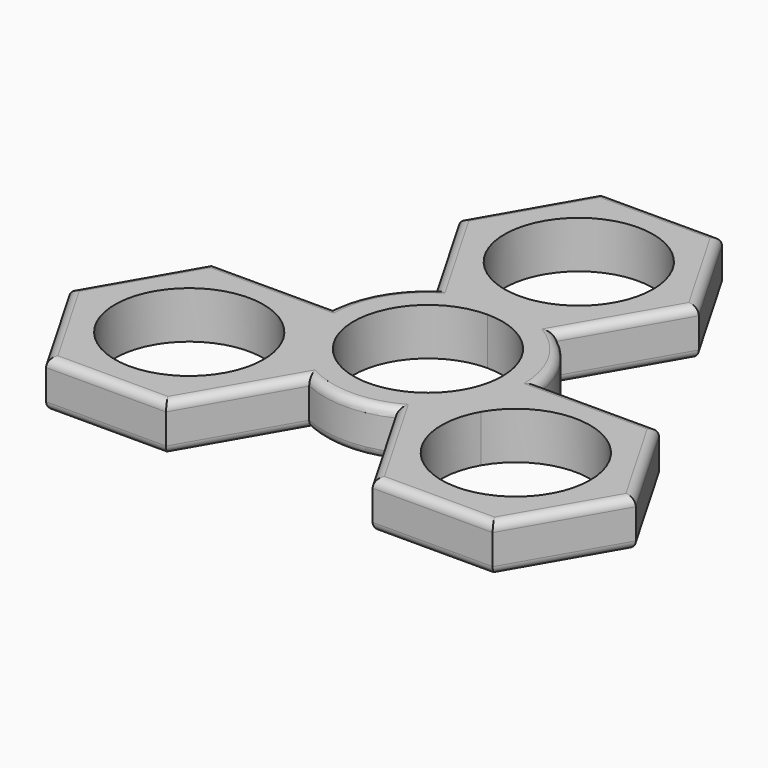
from build123d import *

# Parameters (mm, degrees)
F1_DEPTH      = 6.985
F2_T3_DEPTH   = 24.13
F2_S4_R       = 15.3732097417
F2_T5_DEPTH   = 14
F2_T8_DEPTH   = 24.13
F2_T11_DEPTH  = 24.13
F2_T14_DEPTH  = 24.13
F2_T17_DEPTH  = 24.13
F2_S18_R      = 15.3732097417
F2_T19_DEPTH  = 14
F2_T22_ANGLE  = 73.0101001262
F2_T27_ANGLE  = 73.0101001262
F2_T32_DEPTH  = 24.13
F2_S33_R      = 15.3732097417
F2_T34_DEPTH  = 14
F2_T37_DEPTH  = 24.13
F2_T40_DEPTH  = 24.13
F2_T43_DEPTH  = 24.13
F2_T46_ANGLE  = 73.0101001262
F2_T51_DEPTH  = 24.13
F2_S52_R      = 15.3732097417
F2_T53_DEPTH  = 14
F2_T56_DEPTH  = 24.13
F2_T59_DEPTH  = 24.13
F2_T62_DEPTH  = 24.13
F2_T65_DEPTH  = 24.13
F2_S66_R      = 15.3732097417
F2_T67_DEPTH  = 14
F2_T70_DEPTH  = 24.13
F2_S71_R      = 15.3732097417
F2_T72_DEPTH  = 14
F2_T76_DEPTH  = 24.13
F2_S77_R      = 15.3732097417
F2_T78_DEPTH  = 14
F2_T81_ANGLE  = 73.0101001262
F2_T87_DEPTH  = 24.13
F2_S88_R      = 15.3732097417
F2_T89_DEPTH  = 14
F2_T92_ANGLE  = 73.0101001262
F2_T98_DEPTH  = 24.13
F2_S99_R      = 15.3732097417
F2_T100_DEPTH = 14
F2_T103_ANGLE = 73.0101001262
F2_T109_ANGLE = 73.0101001262
F2_T113_DEPTH = 24.13
F2_S114_R     = 15.3732097417
F2_T115_DEPTH = 14
F2_T120_DEPTH = 24.13
F2_S121_R     = 15.3732097417
F2_T122_DEPTH = 14
F2_T125_ANGLE = 73.0101001262
F2_T131_ANGLE = 73.0101001262
F2_T135_DEPTH = 24.13
F2_S136_R     = 15.3732097417
F2_T137_DEPTH = 14
F3_R          = 1.27


# Not quite as in the source:
# - a fillet or chamfer that OpenCascade refuses, or shapes differently, is made with other operations: its cross-section is extruded or revolved along the edge and cut away or added


with BuildPart() as f1:
    # F0 (on Top) → F1 (new body)
    with BuildSketch(Plane.XY):
        with BuildLine():
            ThreePointArc((0, 11.0109), (7.785882057, 7.785882057), (11.0109, 0))
            ThreePointArc((11.0109, 0), (10.6357126807, -2.8498306237), (9.5357191185, -5.50545))
            Line((9.5357191185, -5.50545), (10.8617497817, -6.2710341604))
            Line((10.8617497817, -6.2710341604), (15.3067497817, 1.4279316793))
            ThreePointArc((15.3067497817, 1.4279316793), (13.313590174, 7.6866048708), (8.89, 12.5420683207))
            Line((8.89, 12.5420683207), (0, 12.5420683207))
            Line((0, 12.5420683207), (0, 11.0109))
        make_face()
        with BuildLine():
            ThreePointArc((-9.5357191185, -5.50545), (-9.5357191185, 5.50545), (0, 11.0109))
            Line((0, 11.0109), (0, 12.5420683207))
            Line((0, 12.5420683207), (-8.89, 12.5420683207))
            ThreePointArc((-8.89, 12.5420683207), (-13.313590174, 7.6866048708), (-15.3067497817, 1.4279316793))
            Line((-15.3067497817, 1.4279316793), (-10.8617497817, -6.2710341604))
            Line((-10.8617497817, -6.2710341604), (-9.5357191185, -5.50545))
        make_face()
        with BuildLine():
            Line((10.8617497817, -6.2710341604), (9.5357191185, -5.50545))
            ThreePointArc((9.5357191185, -5.50545), (0, -11.0109), (-9.5357191185, -5.50545))
            Line((-9.5357191185, -5.50545), (-10.8617497817, -6.2710341604))
            Line((-10.8617497817, -6.2710341604), (-6.4167497817, -13.97))
            ThreePointArc((-6.4167497817, -13.97), (0, -15.3732097417), (6.4167497817, -13.97))
            Line((6.4167497817, -13.97), (10.8617497817, -6.2710341604))
        make_face()
        with BuildLine():
            Line((-8.89, 12.5420683207), (0, 12.5420683207))
            Line((0, 12.5420683207), (0, 15.3732097417))
            ThreePointArc((0, 15.3732097417), (-4.6649614614, 14.648334797), (-8.89, 12.5420683207))
        make_face()
        with BuildLine():
            Line((0, 15.3732097417), (0, 12.5420683207))
            Line((0, 12.5420683207), (8.89, 12.5420683207))
            ThreePointArc((8.89, 12.5420683207), (4.6649614614, 14.648334797), (0, 15.3732097417))
        make_face()
        with BuildLine():
            Line((15.3067497817, 1.4279316793), (10.8617497817, -6.2710341604))
            Line((10.8617497817, -6.2710341604), (13.313590174, -7.6866048708))
            ThreePointArc((13.313590174, -7.6866048708), (14.8493803224, -3.9788794655), (15.3732097417, 0))
            ThreePointArc((15.3732097417, 0), (15.3565857634, 0.7147387297), (15.3067497817, 1.4279316793))
        make_face()
        with BuildLine():
            Line((13.313590174, -7.6866048708), (10.8617497817, -6.2710341604))
            Line((10.8617497817, -6.2710341604), (6.4167497817, -13.97))
            ThreePointArc((6.4167497817, -13.97), (10.3533493266, -11.3641425318), (13.313590174, -7.6866048708))
        make_face()
        with BuildLine():
            Line((-6.4167497817, -13.97), (-10.8617497817, -6.2710341604))
            Line((-10.8617497817, -6.2710341604), (-13.313590174, -7.6866048708))
            ThreePointArc((-13.313590174, -7.6866048708), (-10.3533493266, -11.3641425318), (-6.4167497817, -13.97))
        make_face()
        with BuildLine():
            Line((-13.313590174, -7.6866048708), (-10.8617497817, -6.2710341604))
            Line((-10.8617497817, -6.2710341604), (-15.3067497817, 1.4279316793))
            ThreePointArc((-15.3067497817, 1.4279316793), (-15.018310788, -3.2841922653), (-13.313590174, -7.6866048708))
        make_face()
        with BuildLine():
            ThreePointArc((-8.89, 12.5420683207), (-4.6649614614, 14.648334797), (0, 15.3732097417))
            ThreePointArc((0, 15.3732097417), (4.6649614614, 14.648334797), (8.89, 12.5420683207))
            Line((8.89, 12.5420683207), (17.78, 27.94))
            Line((17.78, 27.94), (8.89, 43.3379316793))
            Line((8.89, 43.3379316793), (-8.89, 43.3379316793))
            Line((-8.89, 43.3379316793), (-17.78, 27.94))
            Line((-17.78, 27.94), (-8.89, 12.5420683207))
        make_face()
        with BuildLine():
            ThreePointArc((11.0109, 27.94), (7.785882057, 20.154117943), (0, 16.9291))
            ThreePointArc((0, 16.9291), (-7.785882057, 35.725882057), (11.0109, 27.94))
        make_face(mode=Mode.SUBTRACT)
        with BuildLine():
            ThreePointArc((15.3732097417, 0), (14.8493803224, -3.9788794655), (13.313590174, -7.6866048708))
            ThreePointArc((13.313590174, -7.6866048708), (10.3533493266, -11.3641425318), (6.4167497817, -13.97))
            Line((6.4167497817, -13.97), (15.3067497817, -29.3679316793))
            Line((15.3067497817, -29.3679316793), (33.0867497817, -29.3679316793))
            Line((33.0867497817, -29.3679316793), (41.9767497817, -13.97))
            Line((41.9767497817, -13.97), (33.0867497817, 1.4279316793))
            Line((33.0867497817, 1.4279316793), (15.3067497817, 1.4279316793))
            ThreePointArc((15.3067497817, 1.4279316793), (15.3565857634, 0.7147387297), (15.3732097417, 0))
        make_face()
        with BuildLine():
            ThreePointArc((35.2076497817, -13.97), (21.346919158, -24.6057126807), (14.6610306632, -8.46455))
            ThreePointArc((14.6610306632, -8.46455), (27.0465804055, -3.3342873193), (35.2076497817, -13.97))
        make_face(mode=Mode.SUBTRACT)
        with BuildLine():
            ThreePointArc((-6.4167497817, -13.97), (-10.3533493266, -11.3641425318), (-13.313590174, -7.6866048708))
            ThreePointArc((-13.313590174, -7.6866048708), (-15.018310788, -3.2841922653), (-15.3067497817, 1.4279316793))
            Line((-15.3067497817, 1.4279316793), (-33.0867497817, 1.4279316793))
            Line((-33.0867497817, 1.4279316793), (-41.9767497817, -13.97))
            Line((-41.9767497817, -13.97), (-33.0867497817, -29.3679316793))
            Line((-33.0867497817, -29.3679316793), (-15.3067497817, -29.3679316793))
            Line((-15.3067497817, -29.3679316793), (-6.4167497817, -13.97))
        make_face()
        with BuildLine():
            ThreePointArc((-13.1858497817, -13.97), (-34.8324624624, -16.8198306237), (-14.6610306632, -8.46455))
            ThreePointArc((-14.6610306632, -8.46455), (-13.5610371011, -11.1201693763), (-13.1858497817, -13.97))
        make_face(mode=Mode.SUBTRACT)
    extrude(amount=F1_DEPTH)

    # F2: fillet of radius 1.27 on 18 edges, made by hand


with BuildPart() as f2_tool1:
    # F2_s2 → F2_t3 (new body)
    with BuildSketch(Plane(origin=(-18.1308748909, 31.4035964967, 0), x_dir=(0, 0, 1), z_dir=(0.5, -0.8660254038, 0))):
        with BuildLine():
            ThreePointArc((5.715, 1.4279316793), (6.6130256121, 1.0559572914), (6.985, 0.1579316793))
            Line((6.985, 0.1579316793), (6.985, 1.4279316793))
            Line((6.985, 1.4279316793), (5.715, 1.4279316793))
        make_face()
    extrude(amount=F2_T3_DEPTH)

    # F2_s4 → F2_t5 (cut, symmetric)
    with BuildSketch(Plane.XY.offset(6.4)):
        Circle(F2_S4_R)
    extrude(amount=F2_T5_DEPTH, both=True, mode=Mode.SUBTRACT)


with BuildPart() as f2_tool6:
    # F2_s7 → F2_t8 (new body)
    with BuildSketch(Plane(origin=(18.1308748909, 31.4035964967, 0), x_dir=(0, 0, 1), z_dir=(-0.5, -0.8660254038, 0))):
        with BuildLine():
            ThreePointArc((5.715, 29.3679316793), (6.6130256121, 28.9959572914), (6.985, 28.0979316793))
            Line((6.985, 28.0979316793), (6.985, 29.3679316793))
            Line((6.985, 29.3679316793), (5.715, 29.3679316793))
        make_face()
    extrude(amount=F2_T8_DEPTH)


with BuildPart() as f2_tool9:
    # F2_s10 → F2_t11 (new body)
    with BuildSketch(Plane.YZ.offset(12.065)):
        with BuildLine():
            ThreePointArc((43.3379316793, 5.715), (42.9659572914, 6.6130256121), (42.0679316793, 6.985))
            Line((42.0679316793, 6.985), (43.3379316793, 6.985))
            Line((43.3379316793, 6.985), (43.3379316793, 5.715))
        make_face()
    extrude(amount=-F2_T11_DEPTH)


with BuildPart() as f2_tool12:
    # F2_s13 → F2_t14 (new body)
    with BuildSketch(Plane(origin=(-6.0658748909, 10.5064035033, 0), x_dir=(0, 0, 1), z_dir=(-0.5, 0.8660254038, 0))):
        with BuildLine():
            ThreePointArc((5.715, 29.3679316793), (6.6130256121, 28.9959572914), (6.985, 28.0979316793))
            Line((6.985, 28.0979316793), (6.985, 29.3679316793))
            Line((6.985, 29.3679316793), (5.715, 29.3679316793))
        make_face()
    extrude(amount=F2_T14_DEPTH)


with BuildPart() as f2_tool15:
    # F2_s16 → F2_t17 (new body)
    with BuildSketch(Plane(origin=(6.0658748909, 10.5064035033, 0), x_dir=(0, 0, 1), z_dir=(0.5, 0.8660254038, 0))):
        with BuildLine():
            ThreePointArc((5.715, 1.4279316793), (6.6130256121, 1.0559572914), (6.985, 0.1579316793))
            Line((6.985, 0.1579316793), (6.985, 1.4279316793))
            Line((6.985, 1.4279316793), (5.715, 1.4279316793))
        make_face()
    extrude(amount=F2_T17_DEPTH)

    # F2_s18 → F2_t19 (cut, symmetric)
    with BuildSketch(Plane.XY.offset(6.4)):
        Circle(F2_S18_R)
    extrude(amount=F2_T19_DEPTH, both=True, mode=Mode.SUBTRACT)


with BuildPart() as f2_tool20:
    # F2_s21 → F2_t22 (revolve)
    with BuildSketch(Plane(origin=(0, 0, 0), x_dir=(0, 0, 1), z_dir=(-0.113290787, -0.9935618741, 0))):
        with BuildLine():
            ThreePointArc((5.715, -15.3732097417), (6.6130256121, -15.0012353538), (6.985, -14.1032097417))
            Line((6.985, -14.1032097417), (6.985, -15.3732097417))
            Line((6.985, -15.3732097417), (5.715, -15.3732097417))
        make_face()
    revolve(axis=Axis((0, 0, 6.985), (0, 0, 1)), revolution_arc=F2_T22_ANGLE)

    split(bisect_by=Plane(origin=(1.2366251091, -0.7139658396, 0), x_dir=(0, 0, 1), z_dir=(0.8660254038, -0.5, 0)), keep=Keep.TOP)

    split(bisect_by=Plane.XZ.offset(-1.4279316793), keep=Keep.BOTTOM)


with BuildPart() as f2_tool25:
    # F2_s26 → F2_t27 (revolve)
    with BuildSketch(Plane(origin=(0, 0, 0), x_dir=(0, 0, 1), z_dir=(0.9170952167, 0.3986682375, 0))):
        with BuildLine():
            ThreePointArc((5.715, -15.3732097417), (6.6130256121, -15.0012353538), (6.985, -14.1032097417))
            Line((6.985, -14.1032097417), (6.985, -15.3732097417))
            Line((6.985, -15.3732097417), (5.715, -15.3732097417))
        make_face()
    revolve(axis=Axis((0, 0, 6.985), (0, 0, 1)), revolution_arc=F2_T27_ANGLE)

    split(bisect_by=Plane(origin=(-1.2366251091, -0.7139658396, 0), x_dir=(0, 0, 1), z_dir=(-0.8660254038, -0.5, 0)), keep=Keep.TOP)

    split(bisect_by=Plane.XZ.offset(-1.4279316793), keep=Keep.BOTTOM)


with BuildPart() as f2_tool30:
    # F2_s31 → F2_t32 (new body)
    with BuildSketch(Plane.YZ.offset(-12.1317497817)):
        with BuildLine():
            ThreePointArc((1.4279316793, 5.715), (1.0559572914, 6.6130256121), (0.1579316793, 6.985))
            Line((0.1579316793, 6.985), (1.4279316793, 6.985))
            Line((1.4279316793, 6.985), (1.4279316793, 5.715))
        make_face()
    extrude(amount=-F2_T32_DEPTH)

    # F2_s33 → F2_t34 (cut, symmetric)
    with BuildSketch(Plane.XY.offset(6.4)):
        Circle(F2_S33_R)
    extrude(amount=F2_T34_DEPTH, both=True, mode=Mode.SUBTRACT)


with BuildPart() as f2_tool35:
    # F2_s36 → F2_t37 (new body)
    with BuildSketch(Plane(origin=(-6.0658748909, -10.5064035033, 0), x_dir=(0, 0, 1), z_dir=(-0.5, -0.8660254038, 0))):
        with BuildLine():
            ThreePointArc((5.715, 29.3679316793), (6.6130256121, 28.9959572914), (6.985, 28.0979316793))
            Line((6.985, 28.0979316793), (6.985, 29.3679316793))
            Line((6.985, 29.3679316793), (5.715, 29.3679316793))
        make_face()
    extrude(amount=F2_T37_DEPTH)


with BuildPart() as f2_tool38:
    # F2_s39 → F2_t40 (new body)
    with BuildSketch(Plane(origin=(-6.0325, 10.4485964967, 0), x_dir=(0, 0, 1), z_dir=(0.5, -0.8660254038, 0))):
        with BuildLine():
            ThreePointArc((5.715, 43.3379316793), (6.6130256121, 42.9659572914), (6.985, 42.0679316793))
            Line((6.985, 42.0679316793), (6.985, 43.3379316793))
            Line((6.985, 43.3379316793), (5.715, 43.3379316793))
        make_face()
    extrude(amount=F2_T40_DEPTH)


with BuildPart() as f2_tool41:
    # F2_s42 → F2_t43 (new body)
    with BuildSketch(Plane.YZ.offset(-36.2617497817)):
        with BuildLine():
            ThreePointArc((-29.3679316793, 5.715), (-28.9959572914, 6.6130256121), (-28.0979316793, 6.985))
            Line((-28.0979316793, 6.985), (-29.3679316793, 6.985))
            Line((-29.3679316793, 6.985), (-29.3679316793, 5.715))
        make_face()
    extrude(amount=F2_T43_DEPTH)


with BuildPart() as f2_tool44:
    # F2_s45 → F2_t46 (revolve)
    with BuildSketch(Plane(origin=(0, 0, 0), x_dir=(0, 0, 1), z_dir=(-0.8038044297, 0.5948936366, 0))):
        with BuildLine():
            ThreePointArc((5.715, -15.3732097417), (6.6130256121, -15.0012353538), (6.985, -14.1032097417))
            Line((6.985, -14.1032097417), (6.985, -15.3732097417))
            Line((6.985, -15.3732097417), (5.715, -15.3732097417))
        make_face()
    revolve(axis=Axis((0, 0, 6.985), (0, 0, 1)), revolution_arc=F2_T46_ANGLE)

    split(bisect_by=Plane(origin=(1.2366251091, -0.7139658396, 0), x_dir=(0, 0, 1), z_dir=(0.8660254038, -0.5, 0)), keep=Keep.TOP)

    split(bisect_by=Plane(origin=(-1.2366251091, -0.7139658396, 0), x_dir=(0, 0, 1), z_dir=(-0.8660254038, -0.5, 0)), keep=Keep.TOP)


with BuildPart() as f2_tool49:
    # F2_s50 → F2_t51 (new body)
    with BuildSketch(Plane(origin=(6.0658748909, -10.5064035033, 0), x_dir=(0, 0, 1), z_dir=(0.5, -0.8660254038, 0))):
        with BuildLine():
            ThreePointArc((5.715, 1.4279316793), (6.6130256121, 1.0559572914), (6.985, 0.1579316793))
            Line((6.985, 0.1579316793), (6.985, 1.4279316793))
            Line((6.985, 1.4279316793), (5.715, 1.4279316793))
        make_face()
    extrude(amount=F2_T51_DEPTH)

    # F2_s52 → F2_t53 (cut, symmetric)
    with BuildSketch(Plane.XY.offset(6.4)):
        Circle(F2_S52_R)
    extrude(amount=F2_T53_DEPTH, both=True, mode=Mode.SUBTRACT)


with BuildPart() as f2_tool54:
    # F2_s55 → F2_t56 (new body)
    with BuildSketch(Plane.YZ.offset(12.1317497817)):
        with BuildLine():
            ThreePointArc((-29.3679316793, 5.715), (-28.9959572914, 6.6130256121), (-28.0979316793, 6.985))
            Line((-28.0979316793, 6.985), (-29.3679316793, 6.985))
            Line((-29.3679316793, 6.985), (-29.3679316793, 5.715))
        make_face()
    extrude(amount=F2_T56_DEPTH)


with BuildPart() as f2_tool57:
    # F2_s58 → F2_t59 (new body)
    with BuildSketch(Plane(origin=(-6.0325, -10.4485964967, 0), x_dir=(0, 0, 1), z_dir=(0.5, 0.8660254038, 0))):
        with BuildLine():
            ThreePointArc((5.715, 43.3379316793), (6.6130256121, 42.9659572914), (6.985, 42.0679316793))
            Line((6.985, 42.0679316793), (6.985, 43.3379316793))
            Line((6.985, 43.3379316793), (5.715, 43.3379316793))
        make_face()
    extrude(amount=F2_T59_DEPTH)


with BuildPart() as f2_tool60:
    # F2_s61 → F2_t62 (new body)
    with BuildSketch(Plane(origin=(18.1308748909, -31.4035964967, 0), x_dir=(0, 0, 1), z_dir=(-0.5, 0.8660254038, 0))):
        with BuildLine():
            ThreePointArc((5.715, 29.3679316793), (6.6130256121, 28.9959572914), (6.985, 28.0979316793))
            Line((6.985, 28.0979316793), (6.985, 29.3679316793))
            Line((6.985, 29.3679316793), (5.715, 29.3679316793))
        make_face()
    extrude(amount=F2_T62_DEPTH)


with BuildPart() as f2_tool63:
    # F2_s64 → F2_t65 (new body)
    with BuildSketch(Plane.YZ.offset(36.2617497817)):
        with BuildLine():
            ThreePointArc((1.4279316793, 5.715), (1.0559572914, 6.6130256121), (0.1579316793, 6.985))
            Line((0.1579316793, 6.985), (1.4279316793, 6.985))
            Line((1.4279316793, 6.985), (1.4279316793, 5.715))
        make_face()
    extrude(amount=-F2_T65_DEPTH)

    # F2_s66 → F2_t67 (cut, symmetric)
    with BuildSketch(Plane.XY.offset(6.4)):
        Circle(F2_S66_R)
    extrude(amount=F2_T67_DEPTH, both=True, mode=Mode.SUBTRACT)


with BuildPart() as f2_tool68:
    # F2_s69 → F2_t70 (new body)
    with BuildSketch(Plane(origin=(-18.1308748909, -31.4035964967, 0), x_dir=(0, 0, 1), z_dir=(0.5, 0.8660254038, 0))):
        with BuildLine():
            ThreePointArc((5.715, 1.4279316793), (6.6130256121, 1.0559572914), (6.985, 0.1579316793))
            Line((6.985, 0.1579316793), (6.985, 1.4279316793))
            Line((6.985, 1.4279316793), (5.715, 1.4279316793))
        make_face()
    extrude(amount=F2_T70_DEPTH)

    # F2_s71 → F2_t72 (cut, symmetric)
    with BuildSketch(Plane.XY.offset(6.4)):
        Circle(F2_S71_R)
    extrude(amount=F2_T72_DEPTH, both=True, mode=Mode.SUBTRACT)


with BuildPart() as f2_tool74:
    # F2_s75 → F2_t76 (new body)
    with BuildSketch(Plane(origin=(-18.1308748909, 31.4035964967, 0), x_dir=(0, 0, 1), z_dir=(0.5, -0.8660254038, 0))):
        with BuildLine():
            ThreePointArc((5.715, 1.4279316793), (6.6130256121, 1.0559572914), (6.985, 0.1579316793))
            Line((6.985, 0.1579316793), (6.985, 1.4279316793))
            Line((6.985, 1.4279316793), (5.715, 1.4279316793))
        make_face()
    extrude(amount=F2_T76_DEPTH)

    # F2_s77 → F2_t78 (intersect, symmetric)
    with BuildSketch(Plane.XY.offset(6.4)):
        Circle(F2_S77_R)
    extrude(amount=F2_T78_DEPTH, both=True, mode=Mode.INTERSECT)


with BuildPart() as f2_tool79:
    # F2_s80 → F2_t81 (revolve)
    with BuildSketch(Plane(origin=(0, 0, 0), x_dir=(0, 0, 1), z_dir=(0.9170952167, 0.3986682375, 0))):
        with BuildLine():
            ThreePointArc((5.715, -15.3732097417), (6.6130256121, -15.0012353538), (6.985, -14.1032097417))
            Line((6.985, -14.1032097417), (6.985, -15.3732097417))
            Line((6.985, -15.3732097417), (5.715, -15.3732097417))
        make_face()
    revolve(axis=Axis((0, 0, 6.985), (0, 0, 1)), revolution_arc=F2_T81_ANGLE)

    split(bisect_by=Plane(origin=(-1.2366251091, -0.7139658396, 0), x_dir=(0, 0, 1), z_dir=(0.8660254038, 0.5, 0)), keep=Keep.TOP)


with BuildPart() as f2_tool74_1:
    add(f2_tool74.part)

    # F2_t83: intersect F2_tool79
    add(f2_tool79.part, mode=Mode.INTERSECT)


with BuildPart() as f2_tool85:
    # F2_s86 → F2_t87 (new body)
    with BuildSketch(Plane(origin=(6.0658748909, 10.5064035033, 0), x_dir=(0, 0, 1), z_dir=(0.5, 0.8660254038, 0))):
        with BuildLine():
            ThreePointArc((5.715, 1.4279316793), (6.6130256121, 1.0559572914), (6.985, 0.1579316793))
            Line((6.985, 0.1579316793), (6.985, 1.4279316793))
            Line((6.985, 1.4279316793), (5.715, 1.4279316793))
        make_face()
    extrude(amount=F2_T87_DEPTH)

    # F2_s88 → F2_t89 (intersect, symmetric)
    with BuildSketch(Plane.XY.offset(6.4)):
        Circle(F2_S88_R)
    extrude(amount=F2_T89_DEPTH, both=True, mode=Mode.INTERSECT)


with BuildPart() as f2_tool90:
    # F2_s91 → F2_t92 (revolve)
    with BuildSketch(Plane(origin=(0, 0, 0), x_dir=(0, 0, 1), z_dir=(-0.113290787, -0.9935618741, 0))):
        with BuildLine():
            ThreePointArc((5.715, -15.3732097417), (6.6130256121, -15.0012353538), (6.985, -14.1032097417))
            Line((6.985, -14.1032097417), (6.985, -15.3732097417))
            Line((6.985, -15.3732097417), (5.715, -15.3732097417))
        make_face()
    revolve(axis=Axis((0, 0, 6.985), (0, 0, 1)), revolution_arc=F2_T92_ANGLE)

    split(bisect_by=Plane(origin=(1.2366251091, -0.7139658396, 0), x_dir=(0, 0, 1), z_dir=(-0.8660254038, 0.5, 0)), keep=Keep.TOP)


with BuildPart() as f2_tool85_1:
    add(f2_tool85.part)

    # F2_t94: intersect F2_tool90
    add(f2_tool90.part, mode=Mode.INTERSECT)


with BuildPart() as f2_tool96:
    # F2_s97 → F2_t98 (new body)
    with BuildSketch(Plane.YZ.offset(36.2617497817)):
        with BuildLine():
            ThreePointArc((1.4279316793, 5.715), (1.0559572914, 6.6130256121), (0.1579316793, 6.985))
            Line((0.1579316793, 6.985), (1.4279316793, 6.985))
            Line((1.4279316793, 6.985), (1.4279316793, 5.715))
        make_face()
    extrude(amount=-F2_T98_DEPTH)

    # F2_s99 → F2_t100 (intersect, symmetric)
    with BuildSketch(Plane.XY.offset(6.4)):
        Circle(F2_S99_R)
    extrude(amount=F2_T100_DEPTH, both=True, mode=Mode.INTERSECT)


with BuildPart() as f2_tool101:
    # F2_s102 → F2_t103 (revolve)
    with BuildSketch(Plane(origin=(0, 0, 0), x_dir=(0, 0, 1), z_dir=(-0.113290787, -0.9935618741, 0))):
        with BuildLine():
            ThreePointArc((5.715, -15.3732097417), (6.6130256121, -15.0012353538), (6.985, -14.1032097417))
            Line((6.985, -14.1032097417), (6.985, -15.3732097417))
            Line((6.985, -15.3732097417), (5.715, -15.3732097417))
        make_face()
    revolve(axis=Axis((0, 0, 6.985), (0, 0, 1)), revolution_arc=F2_T103_ANGLE)

    split(bisect_by=Plane.XZ.offset(-1.4279316793), keep=Keep.TOP)


with BuildPart() as f2_tool96_1:
    add(f2_tool96.part)

    # F2_t105: intersect F2_tool101
    add(f2_tool101.part, mode=Mode.INTERSECT)


with BuildPart() as f2_tool107:
    # F2_s108 → F2_t109 (revolve)
    with BuildSketch(Plane(origin=(0, 0, 0), x_dir=(0, 0, 1), z_dir=(0.9170952167, 0.3986682375, 0))):
        with BuildLine():
            ThreePointArc((5.715, -15.3732097417), (6.6130256121, -15.0012353538), (6.985, -14.1032097417))
            Line((6.985, -14.1032097417), (6.985, -15.3732097417))
            Line((6.985, -15.3732097417), (5.715, -15.3732097417))
        make_face()
    revolve(axis=Axis((0, 0, 6.985), (0, 0, 1)), revolution_arc=F2_T109_ANGLE)

    split(bisect_by=Plane.XZ.offset(-1.4279316793), keep=Keep.TOP)


with BuildPart() as f2_tool111:
    # F2_s112 → F2_t113 (new body)
    with BuildSketch(Plane.YZ.offset(-12.1317497817)):
        with BuildLine():
            ThreePointArc((1.4279316793, 5.715), (1.0559572914, 6.6130256121), (0.1579316793, 6.985))
            Line((0.1579316793, 6.985), (1.4279316793, 6.985))
            Line((1.4279316793, 6.985), (1.4279316793, 5.715))
        make_face()
    extrude(amount=-F2_T113_DEPTH)

    # F2_s114 → F2_t115 (intersect, symmetric)
    with BuildSketch(Plane.XY.offset(6.4)):
        Circle(F2_S114_R)
    extrude(amount=F2_T115_DEPTH, both=True, mode=Mode.INTERSECT)


with BuildPart() as f2_tool107_1:
    add(f2_tool107.part)

    # F2_t116: intersect F2_tool111
    add(f2_tool111.part, mode=Mode.INTERSECT)


with BuildPart() as f2_tool118:
    # F2_s119 → F2_t120 (new body)
    with BuildSketch(Plane(origin=(-18.1308748909, -31.4035964967, 0), x_dir=(0, 0, 1), z_dir=(0.5, 0.8660254038, 0))):
        with BuildLine():
            ThreePointArc((5.715, 1.4279316793), (6.6130256121, 1.0559572914), (6.985, 0.1579316793))
            Line((6.985, 0.1579316793), (6.985, 1.4279316793))
            Line((6.985, 1.4279316793), (5.715, 1.4279316793))
        make_face()
    extrude(amount=F2_T120_DEPTH)

    # F2_s121 → F2_t122 (intersect, symmetric)
    with BuildSketch(Plane.XY.offset(6.4)):
        Circle(F2_S121_R)
    extrude(amount=F2_T122_DEPTH, both=True, mode=Mode.INTERSECT)


with BuildPart() as f2_tool123:
    # F2_s124 → F2_t125 (revolve)
    with BuildSketch(Plane(origin=(0, 0, 0), x_dir=(0, 0, 1), z_dir=(-0.8038044297, 0.5948936366, 0))):
        with BuildLine():
            ThreePointArc((5.715, -15.3732097417), (6.6130256121, -15.0012353538), (6.985, -14.1032097417))
            Line((6.985, -14.1032097417), (6.985, -15.3732097417))
            Line((6.985, -15.3732097417), (5.715, -15.3732097417))
        make_face()
    revolve(axis=Axis((0, 0, 6.985), (0, 0, 1)), revolution_arc=F2_T125_ANGLE)

    split(bisect_by=Plane(origin=(1.2366251091, -0.7139658396, 0), x_dir=(0, 0, 1), z_dir=(-0.8660254038, 0.5, 0)), keep=Keep.TOP)


with BuildPart() as f2_tool118_1:
    add(f2_tool118.part)

    # F2_t127: intersect F2_tool123
    add(f2_tool123.part, mode=Mode.INTERSECT)


with BuildPart() as f2_tool129:
    # F2_s130 → F2_t131 (revolve)
    with BuildSketch(Plane(origin=(0, 0, 0), x_dir=(0, 0, 1), z_dir=(-0.8038044297, 0.5948936366, 0))):
        with BuildLine():
            ThreePointArc((5.715, -15.3732097417), (6.6130256121, -15.0012353538), (6.985, -14.1032097417))
            Line((6.985, -14.1032097417), (6.985, -15.3732097417))
            Line((6.985, -15.3732097417), (5.715, -15.3732097417))
        make_face()
    revolve(axis=Axis((0, 0, 6.985), (0, 0, 1)), revolution_arc=F2_T131_ANGLE)

    split(bisect_by=Plane(origin=(-1.2366251091, -0.7139658396, 0), x_dir=(0, 0, 1), z_dir=(0.8660254038, 0.5, 0)), keep=Keep.TOP)


with BuildPart() as f2_tool133:
    # F2_s134 → F2_t135 (new body)
    with BuildSketch(Plane(origin=(6.0658748909, -10.5064035033, 0), x_dir=(0, 0, 1), z_dir=(0.5, -0.8660254038, 0))):
        with BuildLine():
            ThreePointArc((5.715, 1.4279316793), (6.6130256121, 1.0559572914), (6.985, 0.1579316793))
            Line((6.985, 0.1579316793), (6.985, 1.4279316793))
            Line((6.985, 1.4279316793), (5.715, 1.4279316793))
        make_face()
    extrude(amount=F2_T135_DEPTH)

    # F2_s136 → F2_t137 (intersect, symmetric)
    with BuildSketch(Plane.XY.offset(6.4)):
        Circle(F2_S136_R)
    extrude(amount=F2_T137_DEPTH, both=True, mode=Mode.INTERSECT)


with BuildPart() as f2_tool129_1:
    add(f2_tool129.part)

    # F2_t138: intersect F2_tool133
    add(f2_tool133.part, mode=Mode.INTERSECT)


with BuildPart() as f1_1:
    add(f1.part)

    # F2_t139: cut F2_tool1, F2_tool6, F2_tool9, F2_tool12, F2_tool15, F2_tool20, F2_tool25, F2_tool30, F2_tool35, F2_tool38, F2_tool41, F2_tool44, F2_tool49, F2_tool54, F2_tool57, F2_tool60, F2_tool63, F2_tool68, F2_tool74, F2_tool85, F2_tool96, F2_tool107, F2_tool118, F2_tool129
    add([f2_tool1.part, f2_tool6.part, f2_tool9.part, f2_tool12.part, f2_tool15.part, f2_tool20.part, f2_tool25.part, f2_tool30.part, f2_tool35.part, f2_tool38.part, f2_tool41.part, f2_tool44.part, f2_tool49.part, f2_tool54.part, f2_tool57.part, f2_tool60.part, f2_tool63.part, f2_tool68.part, f2_tool74_1.part, f2_tool85_1.part, f2_tool96_1.part, f2_tool107_1.part, f2_tool118_1.part, f2_tool129_1.part], mode=Mode.SUBTRACT)

    # F3
    f3_edges = [f1_1.edges().sort_by_distance(p)[0] for p in [
        (-24.19675, -29.367932, 0),
        (-10.86175, -21.668966, 0),
        (-37.53175, -21.668966, 0),
        (-37.53175, -6.271034, 0),
        (-24.19675, 1.427932, 0),
        (-13.31359, 7.686605, 0),
        (-13.335, 20.241034, 0),
        (-13.335, 35.638966, 0),
        (0, 43.337932, 0),
        (13.335, 35.638966, 0),
        (13.335, 20.241034, 0),
        (13.31359, 7.686605, 0),
        (24.19675, 1.427932, 0),
        (37.53175, -6.271034, 0),
        (37.53175, -21.668966, 0),
        (24.19675, -29.367932, 0),
        (10.86175, -21.668966, 0),
        (0, -15.37321, 0),
    ]]
    fillet(f3_edges, radius=F3_R)


solid = f1_1.part
